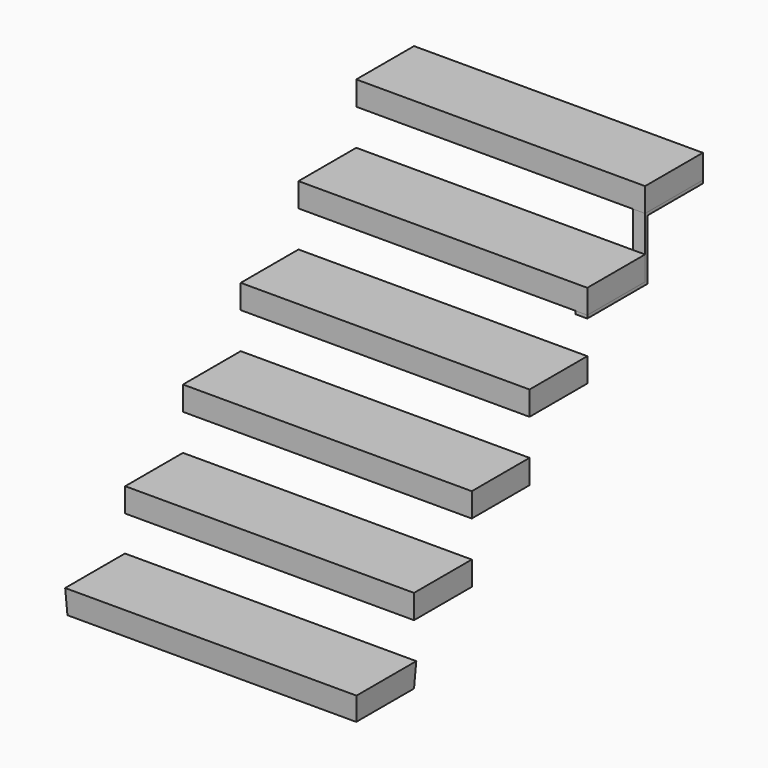
from build123d import *

# Parameters (mm, degrees)
F0_W      = 1219.2
F0_H      = 304.8
F1_DEPTH  = 101.6
F1_TAPER  = -3
F3_W      = 1219.2
F3_H      = 304.8
F4_DEPTH  = 101.6
F6_W      = 1219.2
F6_H      = 304.8
F7_DEPTH  = 101.6
F9_W      = 1219.2
F9_H      = 304.8
F10_DEPTH = 101.6
F12_W     = 1219.2
F12_H     = 304.8
F13_DEPTH = 101.6
F15_W     = 1219.2
F15_H     = 304.8
F16_DEPTH = 101.6
F18_W     = 50.8
F18_H     = 241.3
F19_DEPTH = 12.7
F20_W     = 50.8
F20_H     = 304.8
F21_DEPTH = 12.7
F22_W     = 50.8
F22_H     = 317.5
F23_DEPTH = 12.7


with BuildPart() as f1:
    # F0 (on Top) → F1 (new body)
    with BuildSketch(Plane.XY):
        Rectangle(F0_W, F0_H)
    extrude(amount=F1_DEPTH, taper=F1_TAPER)


with BuildPart() as f4:
    # F3 (on offset) → F4 (new body)
    with BuildSketch(Plane.XY.offset(254)):
        with Locations((0, 304.8)):
            Rectangle(F3_W, F3_H)
    extrude(amount=F4_DEPTH)


with BuildPart() as f7:
    # F6 (on offset) → F7 (new body)
    with BuildSketch(Plane.XY.offset(508)):
        with Locations((0, 609.6)):
            Rectangle(F6_W, F6_H)
    extrude(amount=F7_DEPTH)


with BuildPart() as f10:
    # F9 (on offset) → F10 (new body)
    with BuildSketch(Plane.XY.offset(762)):
        with Locations((0, 914.4)):
            Rectangle(F9_W, F9_H)
    extrude(amount=F10_DEPTH)


with BuildPart() as f13:
    # F12 (on offset) → F13 (new body)
    with BuildSketch(Plane.XY.offset(1016)):
        with Locations((0, 1219.2)):
            Rectangle(F12_W, F12_H)
    extrude(amount=F13_DEPTH)


with BuildPart() as f16:
    # F15 (on offset) → F16 (new body)
    with BuildSketch(Plane.XY.offset(1270)):
        with Locations((0, 1524)):
            Rectangle(F15_W, F15_H)
    extrude(amount=F16_DEPTH)


with BuildPart() as f19:
    # F18 (on offset) → F19 (new body)
    with BuildSketch(Plane.XZ.offset(-1371.6)):
        with Locations((584.2, 1136.65)):
            Rectangle(F18_W, F18_H)
    extrude(amount=-F19_DEPTH)

    # F20 (on offset) → F21 (join)
    with BuildSketch(Plane.XY.offset(1270)):
        with Locations((584.2, 1524)):
            Rectangle(F20_W, F20_H)
    extrude(amount=-F21_DEPTH)

    # F22 (on offset) → F23 (join)
    with BuildSketch(Plane.XY.offset(1016)):
        with Locations((584.2, 1225.55)):
            Rectangle(F22_W, F22_H)
    extrude(amount=-F23_DEPTH)


solid = Compound([f1.part, f4.part, f7.part, f10.part, f13.part, f16.part, f19.part])
